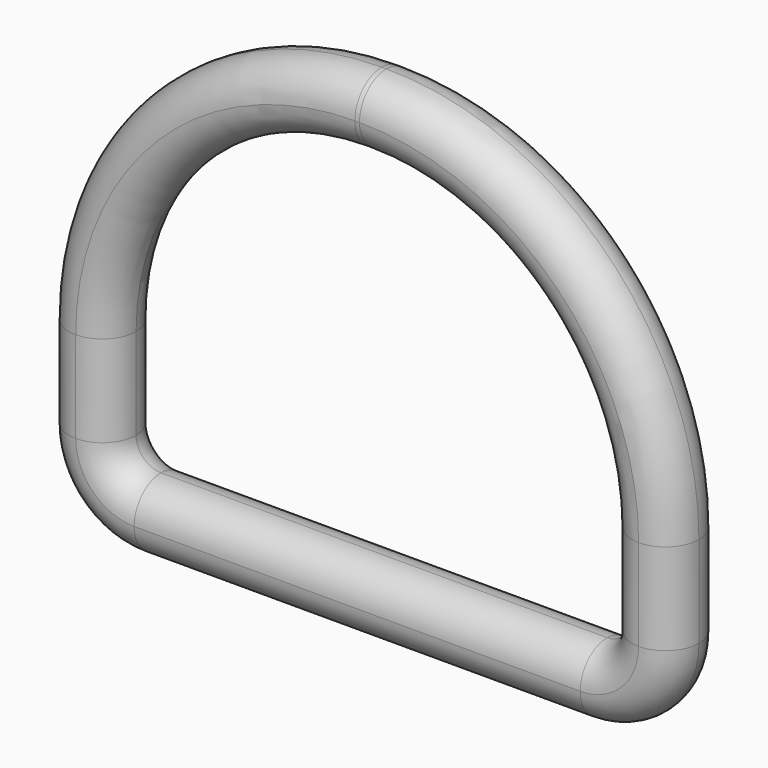
from build123d import *

# Parameters (mm, degrees)
F1_DEPTH = 2.5
F2_R     = 2.49999


# Not quite as in the source:
# - a fillet or chamfer is up to 0.001 mm smaller than in the source, because OpenCascade refuses the exact size


with BuildPart() as f1:
    # F0 (on Front) → F1 (new body, symmetric)
    with BuildSketch(Plane.XZ):
        with BuildLine():
            ThreePointArc((23.5, -4.8265362185), (16.6678157232, 11.6678157232), (0.1734637815, 18.5))
            Line((0.1734637815, 18.5), (-0.1734637815, 18.5))
            ThreePointArc((-0.1734637815, 18.5), (-16.6678157232, 11.6678157232), (-23.5, -4.8265362185))
            Line((-23.5, -4.8265362185), (-23.5, -11.6431219986))
            ThreePointArc((-23.5, -11.6431219986), (-21.4916669312, -16.4916669312), (-16.6431219986, -18.5))
            Line((-16.6431219986, -18.5), (16.6431219986, -18.5))
            ThreePointArc((16.6431219986, -18.5), (21.4916669312, -16.4916669312), (23.5, -11.6431219986))
            Line((23.5, -11.6431219986), (23.5, -4.8265362185))
        make_face()
        with BuildLine():
            Line((-0.1734637815, 13.4999999712), (0.1734637815, 13.4999999712))
            ThreePointArc((0.1734637815, 13.4999999712), (13.1322817969, 8.1322817969), (18.4999999712, -4.8265362185))
            Line((18.4999999712, -4.8265362185), (18.4999999712, -11.6431219986))
            ThreePointArc((18.4999999712, -11.6431219986), (17.9561330049, -12.9561330049), (16.6431219986, -13.4999999712))
            Line((16.6431219986, -13.4999999712), (-16.6431219986, -13.4999999712))
            ThreePointArc((-16.6431219986, -13.4999999712), (-17.9561330049, -12.9561330049), (-18.4999999712, -11.6431219986))
            Line((-18.4999999712, -11.6431219986), (-18.4999999712, -4.8265362185))
            ThreePointArc((-18.4999999712, -4.8265362185), (-13.1322817969, 8.1322817969), (-0.1734637815, 13.4999999712))
        make_face(mode=Mode.SUBTRACT)
    extrude(amount=F1_DEPTH, both=True)

    # F2 (radius 2.5 in the source; OpenCascade refuses exactly that, so slightly less here)
    f2_edges = [f1.edges().sort_by_distance(p)[0] for p in [
        (21.491667, 2.5, -16.491667),
        (23.5, 2.5, -8.234829),
        (16.667816, 2.5, 11.667816),
        (0, 2.5, 18.5),
        (-16.667816, 2.5, 11.667816),
        (-23.5, 2.5, -8.234829),
        (-21.491667, 2.5, -16.491667),
        (0, 2.5, -18.5),
        (0, 2.5, 13.5),
        (13.132282, 2.5, 8.132282),
        (18.5, 2.5, -8.234829),
        (17.956133, 2.5, -12.956133),
        (0, 2.5, -13.5),
        (-17.956133, 2.5, -12.956133),
        (-18.5, 2.5, -8.234829),
        (-13.132282, 2.5, 8.132282),
        (21.491667, -2.5, -16.491667),
        (23.5, -2.5, -8.234829),
        (16.667816, -2.5, 11.667816),
        (0, -2.5, 18.5),
        (-16.667816, -2.5, 11.667816),
        (-23.5, -2.5, -8.234829),
        (-21.491667, -2.5, -16.491667),
        (0, -2.5, -18.5),
        (0, -2.5, 13.5),
        (13.132282, -2.5, 8.132282),
        (18.5, -2.5, -8.234829),
        (17.956133, -2.5, -12.956133),
        (0, -2.5, -13.5),
        (-17.956133, -2.5, -12.956133),
        (-18.5, -2.5, -8.234829),
        (-13.132282, -2.5, 8.132282),
    ]]
    fillet(f2_edges, radius=F2_R)


solid = f1.part
